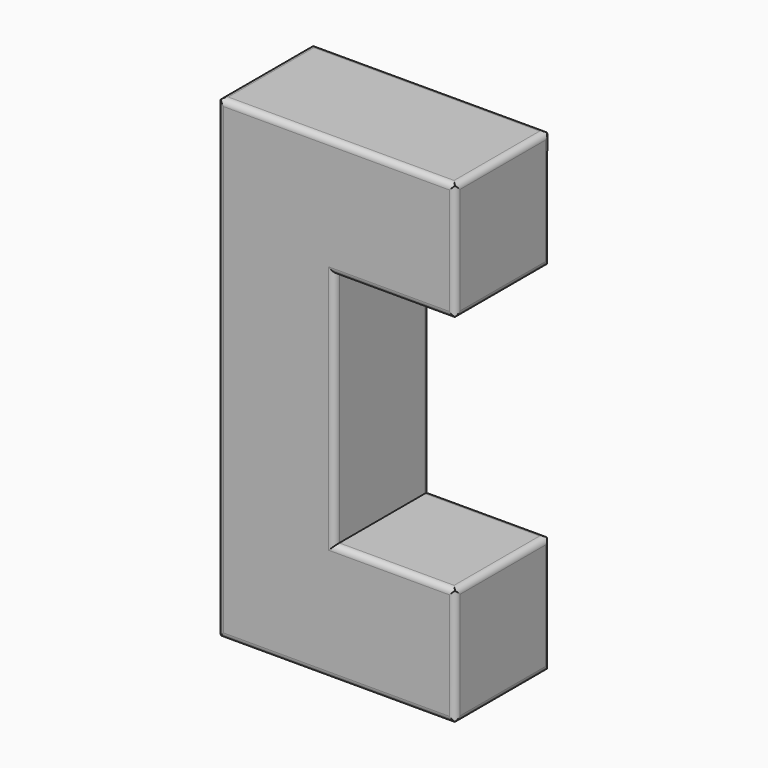
from build123d import *

# Parameters (mm, degrees)
F1_DEPTH    = 10
F2_R        = 0.5
F3_R        = 0.5
F4_T1_DEPTH = 11.5


# Not quite as in the source:
# - a fillet or chamfer that OpenCascade refuses, or shapes differently, is made with other operations: its cross-section is extruded or revolved along the edge and cut away or added


with BuildPart() as f1:
    # F0 (on Front) → F1 (new body)
    with BuildSketch(Plane.XZ):
        Polygon((14.5721812431, 14.7042763403), (-5.4278187569, 14.7042763403), (-5.4278187569, -25.2957236597), (14.5721812431, -25.2957236597), (14.5721812431, -15.2957236597), (4.4125382692, -15.2957236597), (4.4125382692, 4.7042763403), (14.5721812431, 4.7042763403), align=None)
    extrude(amount=F1_DEPTH)

    # F2
    f2_edges = [f1.edges().sort_by_distance(p)[0] for p in [
        (14.572181, -10, 9.704276),
        (4.572181, -10, 14.704276),
        (-5.427819, -10, -5.295724),
        (4.572181, -10, -25.295724),
        (14.572181, -10, -20.295724),
        (9.49236, -10, -15.295724),
        (4.412538, -10, -5.295724),
        (9.49236, -10, 4.704276),
    ]]
    fillet(f2_edges, radius=F2_R)

    # F3
    f3_edges = [f1.edges().sort_by_distance(p)[0] for p in [
        (14.572181, 0, 9.704276),
        (4.572181, 0, 14.704276),
        (-5.427819, 0, -5.295724),
        (4.572181, 0, -25.295724),
        (14.572181, 0, -20.295724),
        (9.49236, 0, -15.295724),
        (4.412538, 0, -5.295724),
        (9.49236, 0, 4.704276),
    ]]
    fillet(f3_edges, radius=F3_R)

    # F4: fillet of radius 0.5 on 16 edges, made by hand

    # F4_s2 → F4_t1 (cut)
    with BuildSketch(Plane.XZ.offset(-0.75)):
        with BuildLine():
            ThreePointArc((14.0721812431, -25.2957236597), (14.4257346337, -25.1492770503), (14.5721812431, -24.7957236597))
            Line((14.5721812431, -24.7957236597), (14.5721812431, -25.2957236597))
            Line((14.5721812431, -25.2957236597), (14.0721812431, -25.2957236597))
        make_face()
        with BuildLine():
            ThreePointArc((14.0721812431, -15.2957236597), (14.4257346337, -15.4421702691), (14.5721812431, -15.7957236597))
            Line((14.5721812431, -15.7957236597), (14.5721812431, -15.2957236597))
            Line((14.5721812431, -15.2957236597), (14.0721812431, -15.2957236597))
        make_face()
        with BuildLine():
            ThreePointArc((-5.4278187569, -24.7957236597), (-5.2813721475, -25.1492770503), (-4.9278187569, -25.2957236597))
            Line((-4.9278187569, -25.2957236597), (-5.4278187569, -25.2957236597))
            Line((-5.4278187569, -25.2957236597), (-5.4278187569, -24.7957236597))
        make_face()
        with BuildLine():
            ThreePointArc((14.5721812431, 5.2042763403), (14.4257346337, 4.8507229497), (14.0721812431, 4.7042763403))
            Line((14.0721812431, 4.7042763403), (14.5721812431, 4.7042763403))
            Line((14.5721812431, 4.7042763403), (14.5721812431, 5.2042763403))
        make_face()
        with BuildLine():
            ThreePointArc((14.5721812431, 14.2042763403), (14.4257346337, 14.5578297309), (14.0721812431, 14.7042763403))
            Line((14.0721812431, 14.7042763403), (14.5721812431, 14.7042763403))
            Line((14.5721812431, 14.7042763403), (14.5721812431, 14.2042763403))
        make_face()
        with BuildLine():
            ThreePointArc((-4.9278187569, 14.7042763403), (-5.2813721475, 14.5578297309), (-5.4278187569, 14.2042763403))
            Line((-5.4278187569, 14.2042763403), (-5.4278187569, 14.7042763403))
            Line((-5.4278187569, 14.7042763403), (-4.9278187569, 14.7042763403))
        make_face()
    extrude(amount=F4_T1_DEPTH, mode=Mode.SUBTRACT)


solid = f1.part
